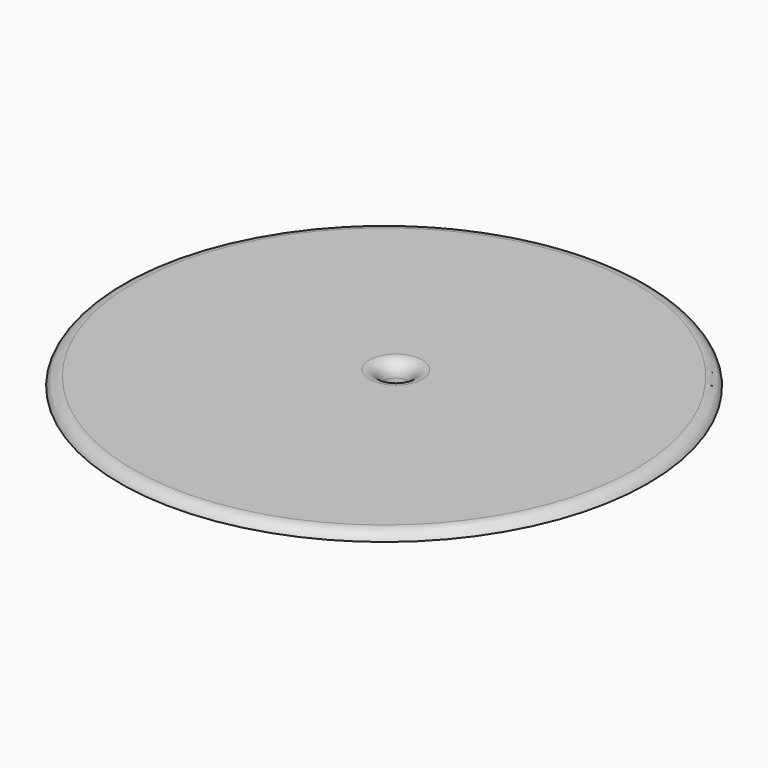
from build123d import *

# Parameters (mm, degrees)
F0_R     = 94.9025273368
F0_R_2   = 4.5
F1_DEPTH = 3
F2_R     = 11
F2_R_2   = 4.5
F3_DEPTH = 30


# Not quite as in the source:
# - a fillet or chamfer that OpenCascade refuses, or shapes differently, is made with other operations: its cross-section is extruded or revolved along the edge and cut away or added


with BuildPart() as f1:
    # F0 (on Top) → F1 (new body)
    with BuildSketch(Plane.XY):
        with Locations((0, -5.2974726632)):
            Circle(F0_R)
        Circle(F0_R_2, mode=Mode.SUBTRACT)
    extrude(amount=F1_DEPTH)

    # F2 (on face) → F3 (join)
    with BuildSketch(Plane(origin=(0, 0, 0), x_dir=(1, 0, 0), z_dir=(0, 0, -1))):
        Circle(F2_R)
        Circle(F2_R_2, mode=Mode.SUBTRACT)
    extrude(amount=F3_DEPTH)

    # F4: fillet of radius 5 on 2 edges, made by hand

    # F4_s1 → F4_t2 (revolve, cut)
    with BuildSketch(Plane.XZ.offset(5.2974726632)):
        with BuildLine():
            ThreePointArc((94.9025273368, 0), (93.0585644294, 2.1833001327), (90.3199516419, 3))
            Line((90.3199516419, 3), (94.9025273368, 3))
            Line((94.9025273368, 3), (94.9025273368, 0))
        make_face()
    revolve(axis=Axis((0, -5.2974726632, 3), (0, 0, 1)), mode=Mode.SUBTRACT)

    # F4_s3 → F4_t4 (revolve, cut)
    with BuildSketch(Plane.XZ):
        with BuildLine():
            ThreePointArc((9.5, 3), (5.9644660941, 1.5355339059), (4.5, -2))
            Line((4.5, -2), (4.5, 3))
            Line((4.5, 3), (9.5, 3))
        make_face()
    revolve(axis=Axis((0, 0, 3), (0, 0, 1)), mode=Mode.SUBTRACT)


solid = f1.part
